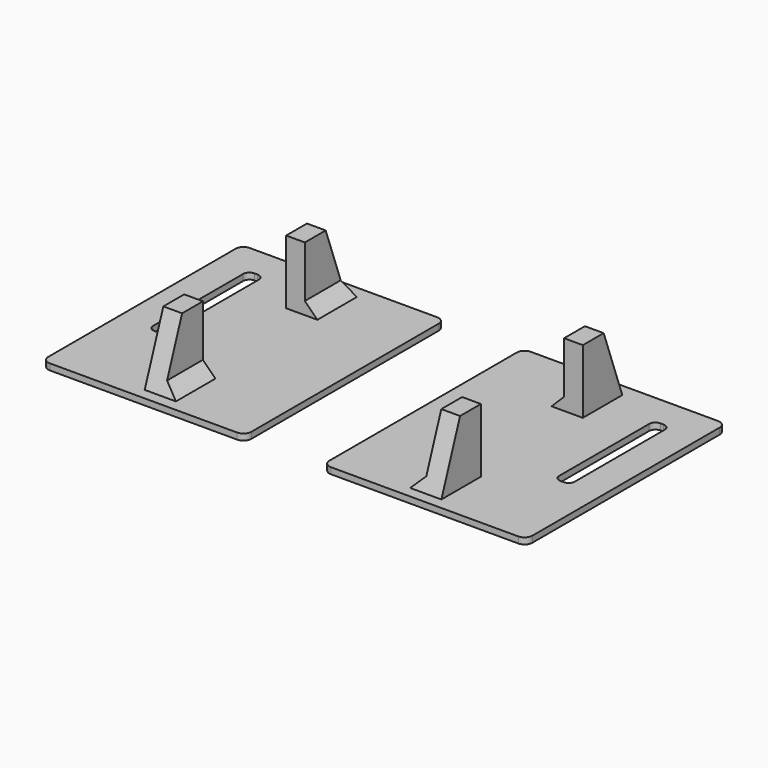
from build123d import *

# Parameters (mm, degrees)
F0_W        = 65
F0_H        = 80
F0_W_2      = 6
F0_H_2      = 7.8
F1_DEPTH    = 2
F2_DEPTH    = 22.5
F3_T4_DEPTH = 6
F3_T9_DEPTH = 6
F4_SIZE     = 4
F5_R        = 2.5
F6_R        = 2


# Not quite as in the source:
# - a fillet or chamfer that OpenCascade refuses, or shapes differently, is made with other operations: its cross-section is extruded or revolved along the edge and cut away or added


with BuildPart() as f1:
    # F0 (on Top) → F1 (new body)
    with BuildSketch(Plane.XY):
        Rectangle(F0_W, F0_H)
        with Locations((0.5000001676, -24.5)):
            Rectangle(F0_W_2, F0_H_2, mode=Mode.SUBTRACT)
        Polygon((-17.5, 10), (-17.5, -10), (-22.5, -10), (-22.5, 30), (-17.5, 30), align=None, mode=Mode.SUBTRACT)
        with Locations((0.5000001676, 24.1)):
            Rectangle(F0_W_2, F0_H_2, mode=Mode.SUBTRACT)
        with Locations((0.5000001676, -24.5)):
            Rectangle(F0_W_2, F0_H_2)
        with Locations((0.5000001676, 24.1)):
            Rectangle(F0_W_2, F0_H_2)
    extrude(amount=F1_DEPTH)

    # F0 (on Top) → F2 (join)
    with BuildSketch(Plane.XY):
        with Locations((0.5000001676, -24.5)):
            Rectangle(F0_W_2, F0_H_2)
        with Locations((0.5000001676, 24.1)):
            Rectangle(F0_W_2, F0_H_2)
    extrude(amount=F2_DEPTH)

    # F3: chamfer of 8 x 21.9798193556 on 2 edges, made by hand


with BuildPart() as f3_tool2:
    # F3_s3 → F3_t4 (new body)
    with BuildSketch(Plane.YZ.offset(3.5000001676)):
        Polygon((-36.4, 2), (-28.4, 23.9798193556), (-28.4, 2), align=None)
    extrude(amount=-F3_T4_DEPTH)

    split(bisect_by=Plane.XY.offset(22.5), keep=Keep.BOTTOM)


with BuildPart() as f1_1:
    add(f1.part)

    # F3_t1: union F3_tool2
    add(f3_tool2.part)


with BuildPart() as f3_tool7:
    # F3_s8 → F3_t9 (new body)
    with BuildSketch(Plane.YZ.offset(-2.4999998324)):
        Polygon((36, 2), (28, 23.9798193556), (28, 2), align=None)
    extrude(amount=F3_T9_DEPTH)

    split(bisect_by=Plane.XY.offset(22.5), keep=Keep.BOTTOM)


with BuildPart() as f1_2:
    add(f1_1.part)

    # F3_t6: union F3_tool7
    add(f3_tool7.part)

    # F4
    f4_edges = [f1_2.edges().sort_by_distance(p)[0] for p in [
        (3.5, -28.5, 2),
        (3.5, 28.1, 2),
    ]]
    chamfer(f4_edges, length=F4_SIZE)

    # F5
    f5_edges = [f1_2.edges().sort_by_distance(p)[0] for p in [
        (-32.5, 40, 1),
        (32.5, 40, 1),
        (32.5, -40, 1),
        (-32.5, -40, 1),
    ]]
    fillet(f5_edges, radius=F5_R)

    # F6
    f6_edges = [f1_2.edges().sort_by_distance(p)[0] for p in [
        (-17.5, 30, 1),
        (-17.5, -10, 1),
        (-22.5, -10, 1),
        (-22.5, 30, 1),
    ]]
    fillet(f6_edges, radius=F6_R)


with BuildPart() as f7_1:
    # F7: instance of F1
    add(f1_2.part.mirror(Plane.YZ))


with BuildPart() as f7_1_1:
    # F8: moved
    add(f7_1.part.moved(Location((90, 0, 0))))


solid = Compound([f1_2.part, f7_1_1.part])
